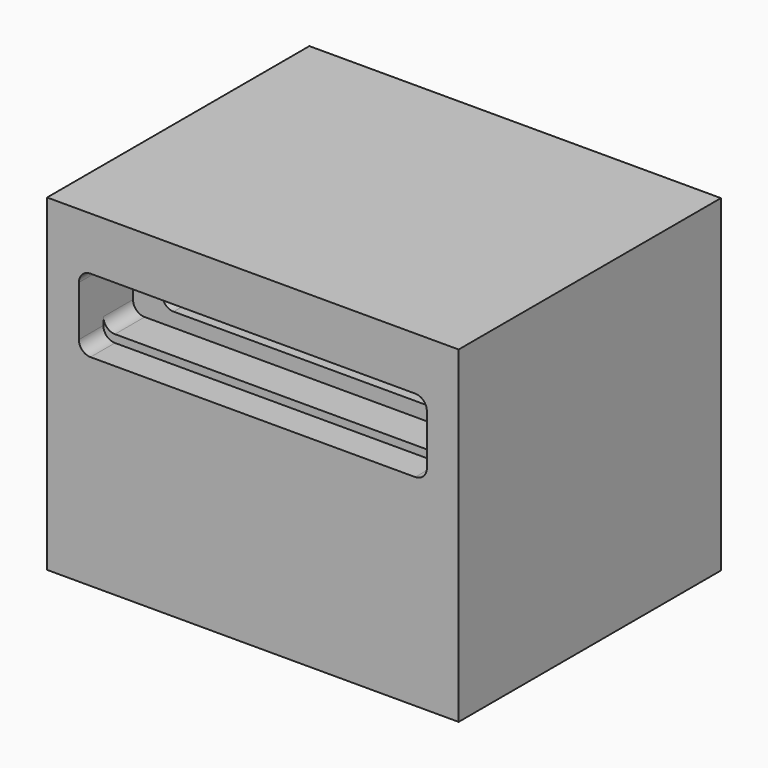
from build123d import *

# Parameters (mm, degrees)
F0_W      = 89.74328
F0_H      = 89.74328
F1_DEPTH  = 112.649
F3_DEPTH  = 8.382
F5_DEPTH  = 10.16
F7_DEPTH  = 10.16
F9_DEPTH  = 25.4
F10_R     = 25.4
F11_DEPTH = 12.7
F12_R     = 19.05
F13_DEPTH = 12.7
F14_R     = 12.7
F15_DEPTH = 42.97172


# Not quite as in the source:
# - a fillet or chamfer that OpenCascade refuses, or shapes differently, is made with other operations: its cross-section is extruded or revolved along the edge and cut away or added


with BuildPart() as f1:
    # F0 (on Right) → F1 (new body)
    with BuildSketch(Plane.YZ):
        with Locations((-0.1941993833, -7.4997466138)):
            Rectangle(F0_W, F0_H)
    extrude(amount=F1_DEPTH)

    # F2 (on face) → F3 (cut)
    with BuildSketch(Plane.XZ.offset(45.0658393833)):
        with BuildLine():
            ThreePointArc((103.9495, 19.7087333862), (103.0195640303, 21.9537974165), (100.7745, 22.8837333862))
            Line((100.7745, 22.8837333862), (11.8745, 22.8837333862))
            ThreePointArc((11.8745, 22.8837333862), (9.6294359697, 21.9537974165), (8.6995, 19.7087333862))
            Line((8.6995, 19.7087333862), (8.6995, 5.9419333862))
            ThreePointArc((8.6995, 5.9419333862), (9.6294359697, 3.6968693559), (11.8745, 2.7669333862))
            Line((11.8745, 2.7669333862), (100.7745, 2.7669333862))
            ThreePointArc((100.7745, 2.7669333862), (103.0195640303, 3.6968693559), (103.9495, 5.9419333862))
            Line((103.9495, 5.9419333862), (103.9495, 19.7087333862))
        make_face()
    extrude(amount=-F3_DEPTH, mode=Mode.SUBTRACT)

    # F4 (on face) → F5 (cut)
    with BuildSketch(Plane.XZ.offset(36.6838393833)):
        with BuildLine():
            ThreePointArc((8.6995, 8.0628333862), (9.6294359697, 5.8177693559), (11.8745, 4.8878333862))
            Line((11.8745, 4.8878333862), (100.7745, 4.8878333862))
            ThreePointArc((100.7745, 4.8878333862), (103.0195640303, 5.8177693559), (103.9495, 8.0628333862))
            Line((103.9495, 8.0628333862), (103.9495, 17.5878333862))
            ThreePointArc((103.9495, 17.5878333862), (103.0195640303, 19.8328974165), (100.7745, 20.7628333862))
            Line((100.7745, 20.7628333862), (11.8745, 20.7628333862))
            ThreePointArc((11.8745, 20.7628333862), (9.6294359697, 19.8328974165), (8.6995, 17.5878333862))
            Line((8.6995, 17.5878333862), (8.6995, 8.0628333862))
        make_face()
    extrude(amount=-F5_DEPTH, mode=Mode.SUBTRACT)

    # F6 (on face) → F7 (cut)
    with BuildSketch(Plane.XZ.offset(26.5238393833)):
        with BuildLine():
            ThreePointArc((16.637, 11.9363333862), (17.5669359697, 9.6912693559), (19.812, 8.7613333862))
            Line((19.812, 8.7613333862), (92.837, 8.7613333862))
            ThreePointArc((92.837, 8.7613333862), (95.0820640303, 9.6912693559), (96.012, 11.9363333862))
            Line((96.012, 11.9363333862), (96.012, 13.7143333862))
            ThreePointArc((96.012, 13.7143333862), (95.0820640303, 15.9593974165), (92.837, 16.8893333862))
            Line((92.837, 16.8893333862), (19.812, 16.8893333862))
            ThreePointArc((19.812, 16.8893333862), (17.5669359697, 15.9593974165), (16.637, 13.7143333862))
            Line((16.637, 13.7143333862), (16.637, 11.9363333862))
        make_face()
    extrude(amount=-F7_DEPTH, mode=Mode.SUBTRACT)

    # F8 (on face) → F9 (cut)
    with BuildSketch(Plane.XZ.offset(16.3638393833)):
        with BuildLine():
            ThreePointArc((88.9, 12.8253333862), (87.9700640303, 15.0703974165), (85.725, 16.0003333862))
            Line((85.725, 16.0003333862), (69.85, 16.0003333862))
            ThreePointArc((69.85, 16.0003333862), (67.6049359697, 15.0703974165), (66.675, 12.8253333862))
            ThreePointArc((66.675, 12.8253333862), (67.6049359697, 10.5802693559), (69.85, 9.6503333862))
            Line((69.85, 9.6503333862), (85.725, 9.6503333862))
            ThreePointArc((85.725, 9.6503333862), (87.9700640303, 10.5802693559), (88.9, 12.8253333862))
        make_face()
    extrude(amount=-F9_DEPTH, mode=Mode.SUBTRACT)

    # F10 (on face) → F11 (cut)
    with BuildSketch(Plane(origin=(0, 0, -52.3713866138), x_dir=(1, 0, 0), z_dir=(0, 0, -1))):
        with Locations((77.7875, -6.5774406167)):
            Circle(F10_R)
    extrude(amount=-F11_DEPTH, mode=Mode.SUBTRACT)

    # F12 (on face) → F13 (cut)
    with BuildSketch(Plane(origin=(0, 0, -39.6713866138), x_dir=(1, 0, 0), z_dir=(0, 0, -1))):
        with Locations((77.7875, -6.5774406167)):
            Circle(F12_R)
    extrude(amount=-F13_DEPTH, mode=Mode.SUBTRACT)

    # F14 (on face) → F15 (cut)
    with BuildSketch(Plane(origin=(0, 0, -26.9713866138), x_dir=(1, 0, 0), z_dir=(0, 0, -1))):
        with Locations((77.7875, -6.5774406167)):
            Circle(F14_R)
    extrude(amount=-F15_DEPTH, mode=Mode.SUBTRACT)

    # F16: fillet of radius 12.90574 on 2 edges, made by hand

    # F16_s1 → F16_t2 (revolve)
    with BuildSketch(Plane.XZ.offset(-6.5774406167)):
        with BuildLine():
            ThreePointArc((103.1875, -50.7880586878), (101.4881153597, -44.3868303291), (96.8375, -39.6713866138))
            Line((96.8375, -39.6713866138), (96.9686148, -39.4490531723))
            ThreePointArc((96.9686148, -39.4490531723), (100.0125, -39.4132718138), (103.1875, -39.4132718138))
            Line((103.1875, -39.4132718138), (103.4456148, -39.6713866138))
            Line((103.4456148, -39.6713866138), (103.4456148, -50.7880586878))
            Line((103.4456148, -50.7880586878), (103.1875, -50.7880586878))
        make_face()
    revolve(axis=Axis((77.7875, 6.5774406167, -39.6713866138), (0, 0, -1)))

    # F16_s3 → F16_t4 (revolve)
    with BuildSketch(Plane.XZ.offset(-6.5774406167)):
        with BuildLine():
            ThreePointArc((96.8375, -38.0880586878), (95.1381153597, -31.6868303291), (90.4875, -26.9713866138))
            Line((90.4875, -26.9713866138), (90.6186148, -26.7490531723))
            ThreePointArc((90.6186148, -26.7490531723), (93.6625, -26.7132718138), (96.8375, -26.7132718138))
            Line((96.8375, -26.7132718138), (97.0956148, -26.9713866138))
            Line((97.0956148, -26.9713866138), (97.0956148, -38.0880586878))
            Line((97.0956148, -38.0880586878), (96.8375, -38.0880586878))
        make_face()
    revolve(axis=Axis((77.7875, 6.5774406167, -26.9713866138), (0, 0, -1)))


solid = f1.part
